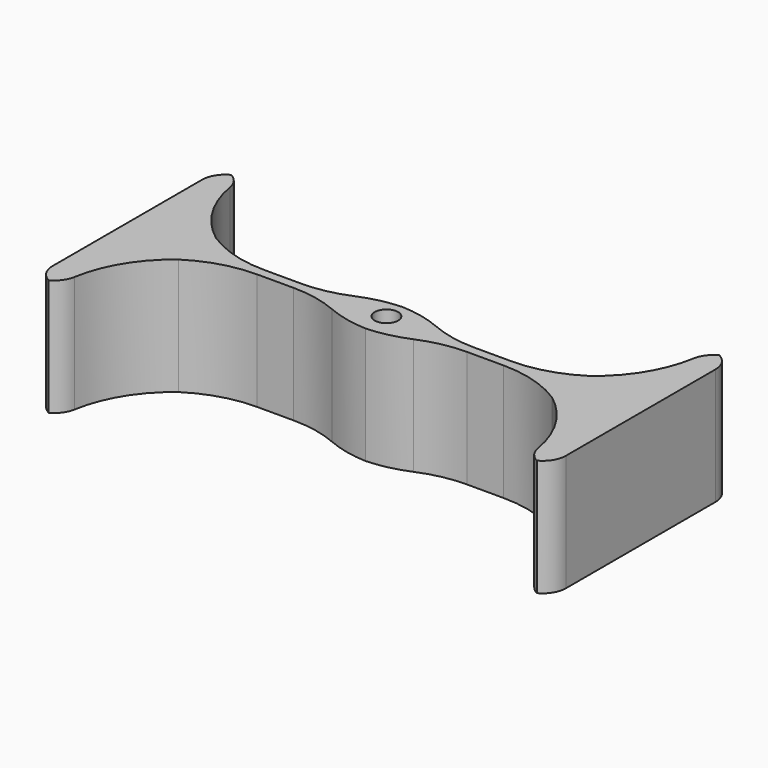
from build123d import *

# Parameters (mm, degrees)
F0_W        = 7
F0_H        = 0.4
F1_DEPTH    = 5
F2_T1_DEPTH = 5
F3_T1_DEPTH = 5
F4_T1_DEPTH = 11.0312579763
F5_T1_DEPTH = 9.5803989155
F5_T3_DEPTH = 10
F6_R        = 0.5
F7_DEPTH    = 5.001


# Not quite as in the source:
# - a fillet or chamfer that OpenCascade refuses, or shapes differently, is made with other operations: its cross-section is extruded or revolved along the edge and cut away or added


with BuildPart() as f1:
    # F0 (on Top) → F1 (new body)
    with BuildSketch(Plane.XY):
        Polygon((9, 4.7017764146), (9, 3.9017764146), (9, 3.5017764146), (9, 2.7017764146), (11, 2.7017764146), (11, 3.5017764146), (11, 3.9017764146), (11, 4.7017764146), align=None)
        with Locations((5.5, 3.7017764146)):
            Rectangle(F0_W, F0_H)
        Polygon((2, 4.7017764146), (0, 4.7017764146), (0, 2.7017764146), (2, 2.7017764146), (2, 3.5017764146), (2, 3.9017764146), align=None)
        Polygon((0, 8.7017764146), (-1, 8.7017764146), (-1, -1.2982235854), (0, -1.2982235854), (0, 2.7017764146), (0, 4.7017764146), align=None)
        with Locations((14.5, 3.7017764146)):
            Rectangle(F0_W, F0_H)
        Polygon((18, 4.7017764146), (18, 3.9017764146), (18, 3.5017764146), (18, 2.7017764146), (20, 2.7017764146), (20, 4.7017764146), align=None)
        Polygon((20, 8.7017764146), (20, 4.7017764146), (20, 2.7017764146), (20, -1.2982235854), (21, -1.2982235854), (21, 8.7017764146), align=None)
    extrude(amount=F1_DEPTH)

    # F2: fillet of radius 5 on 8 edges, made by hand

    # F2_s2 → F2_t1 (join)
    with BuildSketch(Plane.XY):
        with BuildLine():
            ThreePointArc((6.2870680067, 3.5017764146), (7.7012815691, 3.2976079379), (9, 2.7017764145))
            Line((9, 2.7017764145), (9, 3.5017764146))
            Line((9, 3.5017764146), (6.2870680067, 3.5017764146))
        make_face()
        with BuildLine():
            ThreePointArc((15.2870680067, 3.5017764146), (16.7012815691, 3.2976079379), (18, 2.7017764145))
            Line((18, 2.7017764145), (18, 3.5017764146))
            Line((18, 3.5017764146), (15.2870680067, 3.5017764146))
        make_face()
        with BuildLine():
            ThreePointArc((2, 2.7017764145), (3.2987184309, 3.2976079379), (4.7129319933, 3.5017764146))
            Line((4.7129319933, 3.5017764146), (2, 3.5017764146))
            Line((2, 3.5017764146), (2, 2.7017764145))
        make_face()
        with BuildLine():
            ThreePointArc((11, 2.7017764145), (12.2987184309, 3.2976079379), (13.7129319933, 3.5017764146))
            Line((13.7129319933, 3.5017764146), (11, 3.5017764146))
            Line((11, 3.5017764146), (11, 2.7017764145))
        make_face()
        with BuildLine():
            ThreePointArc((13.7129319933, 3.9017764146), (12.2987184309, 4.1059448912), (11, 4.7017764146))
            Line((11, 4.7017764146), (11, 3.9017764146))
            Line((11, 3.9017764146), (13.7129319933, 3.9017764146))
        make_face()
        with BuildLine():
            ThreePointArc((4.7129319933, 3.9017764146), (3.2987184309, 4.1059448912), (2, 4.7017764146))
            Line((2, 4.7017764146), (2, 3.9017764146))
            Line((2, 3.9017764146), (4.7129319933, 3.9017764146))
        make_face()
        with BuildLine():
            ThreePointArc((9, 4.7017764146), (7.7012815691, 4.1059448912), (6.2870680067, 3.9017764146))
            Line((6.2870680067, 3.9017764146), (9, 3.9017764146))
            Line((9, 3.9017764146), (9, 4.7017764146))
        make_face()
        with BuildLine():
            ThreePointArc((18, 4.7017764146), (16.7012815691, 4.1059448912), (15.2870680067, 3.9017764146))
            Line((15.2870680067, 3.9017764146), (18, 3.9017764146))
            Line((18, 3.9017764146), (18, 4.7017764146))
        make_face()
    extrude(amount=F2_T1_DEPTH)

    # F3: fillet of radius 5 on 4 edges, made by hand

    # F3_s2 → F3_t1 (join)
    with BuildSketch(Plane.XY):
        with BuildLine():
            ThreePointArc((20, 8.7017764146), (19.472135955, 6.4657084371), (18, 4.7017764146))
            Line((18, 4.7017764146), (20, 4.7017764146))
            Line((20, 4.7017764146), (20, 8.7017764146))
        make_face()
        with BuildLine():
            ThreePointArc((2, 4.7017764146), (0.527864045, 6.4657084371), (0, 8.7017764146))
            Line((0, 8.7017764146), (0, 4.7017764146))
            Line((0, 4.7017764146), (2, 4.7017764146))
        make_face()
        with BuildLine():
            ThreePointArc((0, -1.2982235854), (0.527864045, 0.9378443921), (2, 2.7017764146))
            Line((2, 2.7017764146), (0, 2.7017764146))
            Line((0, 2.7017764146), (0, -1.2982235854))
        make_face()
        with BuildLine():
            ThreePointArc((18, 2.7017764146), (19.472135955, 0.9378443921), (20, -1.2982235854))
            Line((20, -1.2982235854), (20, 2.7017764146))
            Line((20, 2.7017764146), (18, 2.7017764146))
        make_face()
    extrude(amount=F3_T1_DEPTH)

    # F4: fillet of radius 5 on 4 edges, made by hand

    # F4_s2 → F4_t1 (cut)
    with BuildSketch(Plane.XY.offset(-3.0156289881)):
        with BuildLine():
            ThreePointArc((11.7533401991, 4.3017764145), (10.7937484048, 4.6007559001), (9.7937484047, 4.7017764146))
            Line((9.7937484047, 4.7017764146), (11, 4.7017764146))
            ThreePointArc((11, 4.7017764146), (11.3681250426, 4.4856830772), (11.7533401991, 4.3017764145))
        make_face()
        with BuildLine():
            ThreePointArc((8.2466598009, 4.3017764145), (9.2062515952, 4.6007559001), (10.2062515953, 4.7017764146))
            Line((10.2062515953, 4.7017764146), (9, 4.7017764146))
            ThreePointArc((9, 4.7017764146), (8.6318749574, 4.4856830772), (8.2466598009, 4.3017764145))
        make_face()
        with BuildLine():
            ThreePointArc((9.7937484048, 2.7017764146), (10.7937484048, 2.802796929), (11.7533401991, 3.1017764146))
            ThreePointArc((11.7533401991, 3.1017764146), (11.3681250426, 2.9178697519), (11, 2.7017764146))
            Line((11, 2.7017764146), (9.7937484048, 2.7017764146))
        make_face()
        with BuildLine():
            ThreePointArc((8.2466598009, 3.1017764146), (9.2062515952, 2.802796929), (10.2062515952, 2.7017764146))
            Line((10.2062515952, 2.7017764146), (9, 2.7017764146))
            ThreePointArc((9, 2.7017764146), (8.6318749574, 2.9178697519), (8.2466598009, 3.1017764146))
        make_face()
    extrude(amount=F4_T1_DEPTH, mode=Mode.SUBTRACT)

    # F5: fillet of radius 1 on 8 edges, made by hand

    # F5_s2 → F5_t1 (cut)
    with BuildSketch(Plane.XY.offset(-2.2901994577)):
        with BuildLine():
            ThreePointArc((19.9300664859, 7.8684430812), (20.2705825587, 8.4655390304), (20.9160797831, 8.7017764146))
            Line((20.9160797831, 8.7017764146), (20, 8.7017764146))
            ThreePointArc((20, 8.7017764146), (19.9824859473, 8.2836451132), (19.9300664859, 7.8684430812))
        make_face()
        with BuildLine():
            ThreePointArc((20.9160797831, -1.2982235854), (20.2705825587, -1.0619862013), (19.9300664859, -0.4648902521))
            ThreePointArc((19.9300664859, -0.4648902521), (19.9824859473, -0.880092284), (20, -1.2982235854))
            Line((20, -1.2982235854), (20.9160797831, -1.2982235854))
        make_face()
        with BuildLine():
            ThreePointArc((-0.9160797831, 8.7017764146), (-0.2705825587, 8.4655390304), (0.0699335141, 7.8684430812))
            ThreePointArc((0.0699335141, 7.8684430812), (0.0175140527, 8.2836451132), (0, 8.7017764146))
            Line((0, 8.7017764146), (-0.9160797831, 8.7017764146))
        make_face()
        with BuildLine():
            ThreePointArc((0.0699335141, -0.4648902521), (-0.2705825587, -1.0619862013), (-0.9160797831, -1.2982235854))
            Line((-0.9160797831, -1.2982235854), (0, -1.2982235854))
            ThreePointArc((0, -1.2982235854), (0.0175140527, -0.880092284), (0.0699335141, -0.4648902521))
        make_face()
    extrude(amount=F5_T1_DEPTH, mode=Mode.SUBTRACT)

    # F5_s4 → F5_t3 (cut)
    with BuildSketch(Plane.XY.offset(-2.5)):
        with BuildLine():
            ThreePointArc((20, 8.7017764146), (20.7071067812, 8.4088831957), (21, 7.7017764146))
            Line((21, 7.7017764146), (21, 8.7017764146))
            Line((21, 8.7017764146), (20, 8.7017764146))
        make_face()
        with BuildLine():
            ThreePointArc((21, -0.2982235854), (20.7071067812, -1.0053303666), (20, -1.2982235854))
            Line((20, -1.2982235854), (21, -1.2982235854))
            Line((21, -1.2982235854), (21, -0.2982235854))
        make_face()
        with BuildLine():
            ThreePointArc((-1, 7.7017764146), (-0.7071067812, 8.4088831957), (0, 8.7017764146))
            Line((0, 8.7017764146), (-1, 8.7017764146))
            Line((-1, 8.7017764146), (-1, 7.7017764146))
        make_face()
        with BuildLine():
            ThreePointArc((0, -1.2982235854), (-0.7071067812, -1.0053303666), (-1, -0.2982235854))
            Line((-1, -0.2982235854), (-1, -1.2982235854))
            Line((-1, -1.2982235854), (0, -1.2982235854))
        make_face()
    extrude(amount=F5_T3_DEPTH, mode=Mode.SUBTRACT)

    # F6 (on face) → F7 (cut, through all)
    with BuildSketch(Plane.XY.offset(5)):
        with Locations((10, 3.8341005302)):
            Circle(F6_R)
    extrude(amount=-F7_DEPTH, mode=Mode.SUBTRACT)


solid = f1.part
